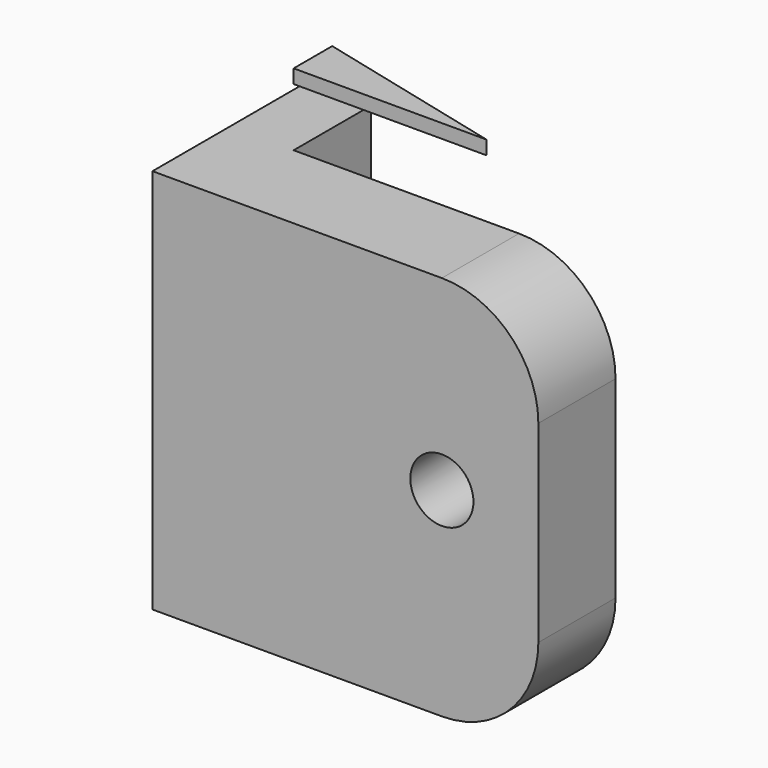
from build123d import *

# Parameters (mm, degrees)
F1_DEPTH = 152.4
F2_R     = 12.4654374507
F3_DEPTH = 41.8860476801
F4_R     = 38.1
F5_R     = 38.1
F8_DEPTH = 5.4713543504


# Not quite as in the source:
# - a pattern or mirror of a feature is missing from the dataset's text; its kind, count and spacing are read off the source's solid


with BuildPart() as f1:
    # F0 (on Top) → F1 (new body)
    with BuildSketch(Plane.XY):
        Polygon((-64.8825142378, 34.3149523199), (-90.1543280485, 34.3149523199), (-90.1543280485, -41.8850476801), (62.2456719515, -41.8850476801), (62.2456719515, -3.7850476801), (-64.8825142378, -3.7850476801), align=None)
    extrude(amount=F1_DEPTH)

    # F2 (on Front) → F3 (cut, through all)
    with BuildSketch(Plane.XZ):
        with Locations((24.1456719515, 78.66833359)):
            Circle(F2_R)
    extrude(amount=F3_DEPTH, mode=Mode.SUBTRACT)

    # F4
    f4_edges = [f1.edges().sort_by_distance(p)[0] for p in [
        (62.245672, -22.835048, 152.4),
    ]]
    fillet(f4_edges, radius=F4_R)

    # F5
    f5_edges = [f1.edges().sort_by_distance(p)[0] for p in [
        (62.245672, -22.835048, 0),
    ]]
    fillet(f5_edges, radius=F5_R)

    # F7 (on offset) → F8 (join)
    with BuildSketch(Plane.XY.offset(44.45)):
        Polygon((-64.8825142378, -3.7850476801), (11.3174857622, -3.7850476801), (-64.8825142378, 15.2649523199), align=None)
    f8 = extrude(amount=-F8_DEPTH)

    # F8_copies: F8 across plane
    add(f8.mirror(Plane.XY.offset(109.927885)))


solid = f1.part
